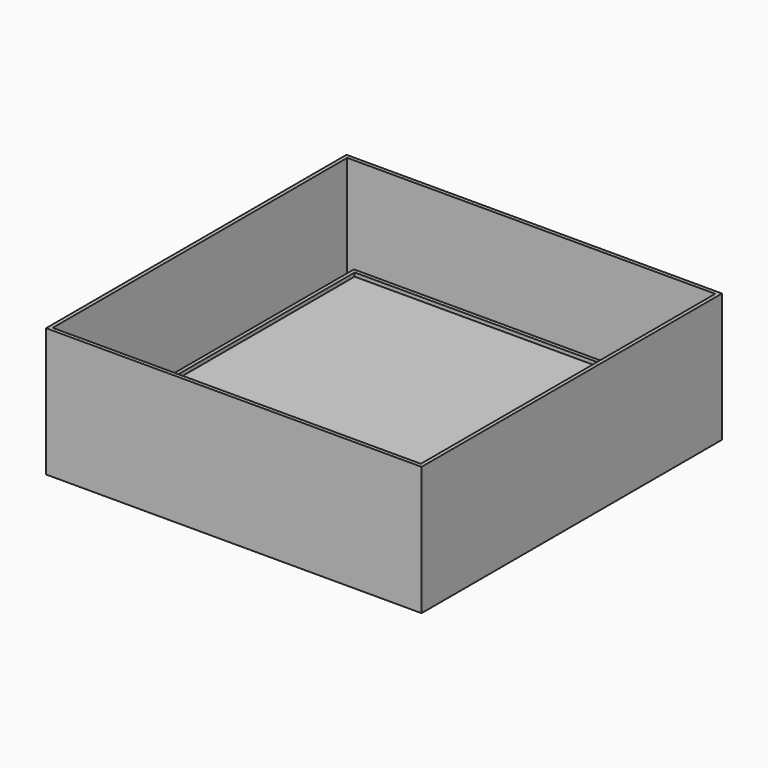
from build123d import *

# Parameters (mm, degrees)
F0_W     = 102
F0_H     = 102
F1_DEPTH = 4
F2_W     = 102
F2_H     = 102
F2_W_2   = 100
F2_H_2   = 100
F3_DEPTH = 35
F4_W     = 81.75
F4_H     = 81.75
F4_W_2   = 79.75
F4_H_2   = 79.75
F5_DEPTH = 15
F7_DEPTH = 10


# Not quite as in the source:
# - a feature names something its author has since deleted; it is built from what else it names


with BuildPart() as f1:
    # F0 (on Top) → F1 (new body)
    with BuildSketch(Plane.XY):
        Rectangle(F0_W, F0_H)
    extrude(amount=F1_DEPTH)

    # F2 (on Top) → F3 (join)
    with BuildSketch(Plane.XY):
        Rectangle(F2_W, F2_H)
        Rectangle(F2_W_2, F2_H_2, mode=Mode.SUBTRACT)
    extrude(amount=F3_DEPTH)

    # F4 (on Top) → F5 (join)
    with BuildSketch(Plane.XY):
        Rectangle(F4_W, F4_H)
        Rectangle(F4_W_2, F4_H_2, mode=Mode.SUBTRACT)
    extrude(amount=F5_DEPTH)

    # F6: union 

    # F7 (add): a face of the model
    f7_faces = [f1.faces().sort_by_distance(p)[0] for p in [
        (0, 0, 4),
    ]]
    extrude(f7_faces, amount=F7_DEPTH)


solid = f1.part
